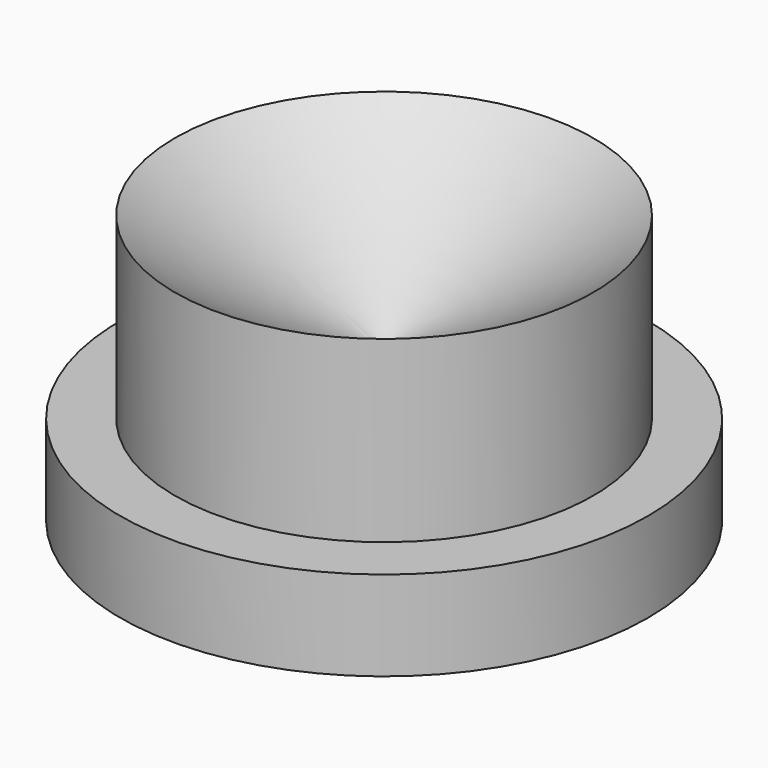
from build123d import *

# Parameters (mm, degrees)
F2_R     = 8.8318475898
F2_R_2   = 7
F3_DEPTH = 3


with BuildPart() as f1:
    # F0 (on Front) → F1 (revolve)
    with BuildSketch(Plane.XZ):
        with BuildLine():
            Line((-56.8012516619, 5.9856966478), (-56.8012516619, 0))
            Line((-56.8012516619, 0), (-49.8012516619, 0))
            Line((-49.8012516619, 0), (-49.8012516619, 2))
            ThreePointArc((-49.8012516619, 2), (-53.4082810787, 3.8048746811), (-56.8012516619, 5.9856966478))
        make_face()
    revolve(axis=Axis((-49.8012516619, 0, 1), (0, 0, -1)))

    # F2 (on face) → F3 (join)
    with BuildSketch(Plane(origin=(0, 0, 0), x_dir=(1, 0, 0), z_dir=(0, 0, -1))):
        with Locations((-49.8012516619, 0)):
            Circle(F2_R)
        with Locations((-49.8012516619, 0)):
            Circle(F2_R_2, mode=Mode.SUBTRACT)
        with Locations((-49.8012516619, 0)):
            Circle(F2_R_2)
    extrude(amount=F3_DEPTH)


solid = f1.part
